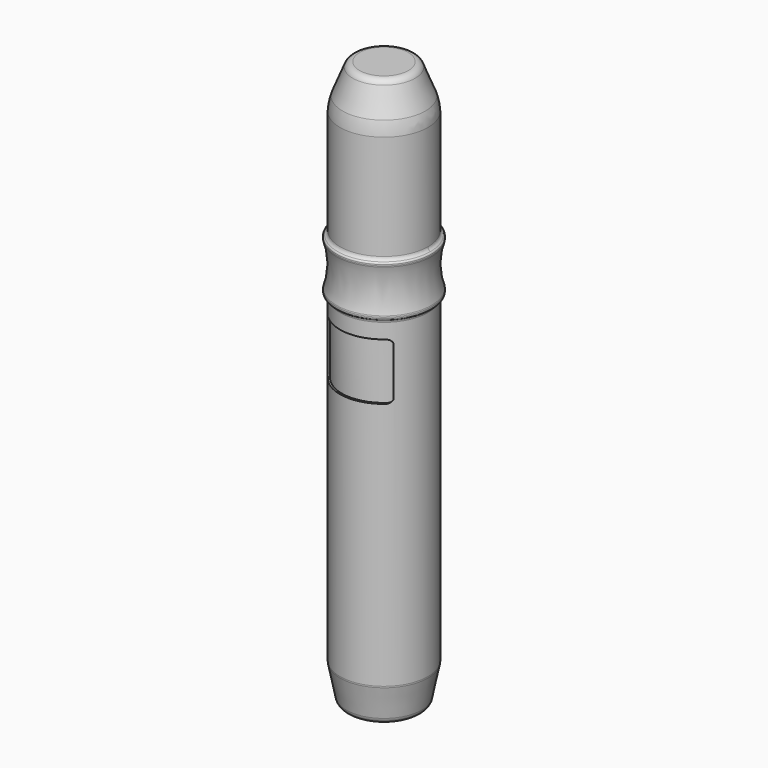
from build123d import *

# Parameters (mm, degrees)
F0_R          = 12
F1_DEPTH      = 154
F2_SIZE2      = 2
F2_SIZE       = 10
F3_SIZE2      = 10
F3_SIZE       = 4
F6_R          = 1
F7_R          = 10
F8_R          = 2
F11_DEPTH     = 15.5
F12_T4_DEPTH  = 7.2783434016
F12_S5_R      = 12
F12_T6_DEPTH  = 5
F12_T10_DEPTH = 7.2783434016
F12_S11_R     = 12
F12_T12_DEPTH = 5
F12_T16_DEPTH = 7.2783434016
F12_S17_R     = 12
F12_T18_DEPTH = 5
F12_T22_DEPTH = 7.2783434016
F12_S23_R     = 12
F12_T24_DEPTH = 5


# Not quite as in the source:
# - a fillet or chamfer that OpenCascade refuses, or shapes differently, is made with other operations: its cross-section is extruded or revolved along the edge and cut away or added
# - a feature names something its author has since deleted; it is built from what else it names


with BuildPart() as f1:
    # F0 (on Top) → F1 (new body)
    with BuildSketch(Plane.XY):
        Circle(F0_R)
    extrude(amount=F1_DEPTH)

    # F2
    f2_edges = [f1.edges().sort_by_distance(p)[0] for p in [
        (-12, 0, 0),
    ]]
    f2_side = f1.faces().sort_by_distance((-12, 0, 77))[0]
    chamfer(f2_edges, length=F2_SIZE, length2=F2_SIZE2, reference=f2_side)

    # F3
    f3_edges = [f1.edges().sort_by_distance(p)[0] for p in [
        (-12, 0, 154),
    ]]
    f3_side = f1.faces().sort_by_distance((0, 0, 154))[0]
    chamfer(f3_edges, length=F3_SIZE, length2=F3_SIZE2, reference=f3_side)

    # F4 (on Front) → F5 (revolve)
    with BuildSketch(Plane.XZ):
        with BuildLine():
            Line((0, 98.5), (0, 112.5))
            Line((0, 112.5), (-12.5, 112.5))
            ThreePointArc((-12.5, 112.5), (-12.8535533906, 112.3535533906), (-13, 112))
            Line((-13, 112), (-13, 111.5))
            ThreePointArc((-13, 111.5), (-12, 105.5), (-13, 99.5))
            Line((-13, 99.5), (-13, 99))
            ThreePointArc((-13, 99), (-12.8535533906, 98.6464466094), (-12.5, 98.5))
            Line((-12.5, 98.5), (0, 98.5))
        make_face()
    revolve(axis=Axis((0, 0, 105.5), (0, 0, 1)))

    # F6
    f6_edges = [f1.edges().sort_by_distance(p)[0] for p in [
        (-12, 0, 112.5),
        (-12, 0, 98.5),
        (13, 0, 99.5),
        (13, 0, 111.5),
    ]]
    fillet(f6_edges, radius=F6_R)

    # F7
    f7_edges = [f1.edges().sort_by_distance(p)[0] for p in [
        (-12, 0, 144),
    ]]
    fillet(f7_edges, radius=F7_R)

    # F8
    f8_edges = [f1.edges().sort_by_distance(p)[0] for p in [
        (-8, 0, 154),
        (-12, 0, 10),
        (-10, 0, 0),
    ]]
    fillet(f8_edges, radius=F8_R)

    # F10 (on offset) → F11 (cut)
    with BuildSketch(Plane(origin=(0, 0, 78), x_dir=(1, 0, 0), z_dir=(0, 0, -1))):
        with BuildLine():
            ThreePointArc((-9, 7.1589105316), (0, 11.5), (9, 7.1589105316))
            Line((9, 7.1589105316), (9, 7.9372539332))
            ThreePointArc((9, 7.9372539332), (0, 12), (-9, 7.9372539332))
            Line((-9, 7.9372539332), (-9, 7.1589105316))
        make_face()
    extrude(amount=-F11_DEPTH, mode=Mode.SUBTRACT)

    # F12: fillet of radius 1.3 on 4 edges, made by hand


with BuildPart() as f12_tool2:
    # F12_s3 → F12_t4 (new body)
    with BuildSketch(Plane.XZ.offset(11.1872539332)):
        with BuildLine():
            ThreePointArc((-9, 92.2), (-8.6192388155, 93.1192388155), (-7.7, 93.5))
            Line((-7.7, 93.5), (-9, 93.5))
            Line((-9, 93.5), (-9, 92.2))
        make_face()
    extrude(amount=-F12_T4_DEPTH)

    # F12_s5 → F12_t6 (intersect, symmetric)
    with BuildSketch(Plane.XY.offset(92.8)):
        Circle(F12_S5_R)
    extrude(amount=F12_T6_DEPTH, both=True, mode=Mode.INTERSECT)


with BuildPart() as f1_1:
    add(f1.part)

    # F12_t1: union F12_tool2
    add(f12_tool2.part)


with BuildPart() as f12_tool8:
    # F12_s9 → F12_t10 (new body)
    with BuildSketch(Plane.XZ.offset(3.9089105316)):
        with BuildLine():
            ThreePointArc((7.7, 93.5), (8.6192388155, 93.1192388155), (9, 92.2))
            Line((9, 92.2), (9, 93.5))
            Line((9, 93.5), (7.7, 93.5))
        make_face()
    extrude(amount=F12_T10_DEPTH)

    # F12_s11 → F12_t12 (intersect, symmetric)
    with BuildSketch(Plane.XY.offset(92.8)):
        Circle(F12_S11_R)
    extrude(amount=F12_T12_DEPTH, both=True, mode=Mode.INTERSECT)


with BuildPart() as f1_2:
    add(f1_1.part)

    # F12_t7: union F12_tool8
    add(f12_tool8.part)


with BuildPart() as f12_tool14:
    # F12_s15 → F12_t16 (new body)
    with BuildSketch(Plane.XZ.offset(3.9089105316)):
        with BuildLine():
            ThreePointArc((7.7, 78), (8.6192388155, 78.3807611845), (9, 79.3))
            Line((9, 79.3), (9, 78))
            Line((9, 78), (7.7, 78))
        make_face()
    extrude(amount=F12_T16_DEPTH)

    # F12_s17 → F12_t18 (intersect, symmetric)
    with BuildSketch(Plane.XY.offset(78.7)):
        Circle(F12_S17_R)
    extrude(amount=F12_T18_DEPTH, both=True, mode=Mode.INTERSECT)


with BuildPart() as f1_3:
    add(f1_2.part)

    # F12_t13: union F12_tool14
    add(f12_tool14.part)


with BuildPart() as f12_tool20:
    # F12_s21 → F12_t22 (new body)
    with BuildSketch(Plane.XZ.offset(11.1872539332)):
        with BuildLine():
            ThreePointArc((-7.7, 78), (-8.6192388155, 78.3807611845), (-9, 79.3))
            Line((-9, 79.3), (-9, 78))
            Line((-9, 78), (-7.7, 78))
        make_face()
    extrude(amount=-F12_T22_DEPTH)

    # F12_s23 → F12_t24 (intersect, symmetric)
    with BuildSketch(Plane.XY.offset(78.7)):
        Circle(F12_S23_R)
    extrude(amount=F12_T24_DEPTH, both=True, mode=Mode.INTERSECT)


with BuildPart() as f1_4:
    add(f1_3.part)

    # F12_t19: union F12_tool20
    add(f12_tool20.part)


solid = f1_4.part
